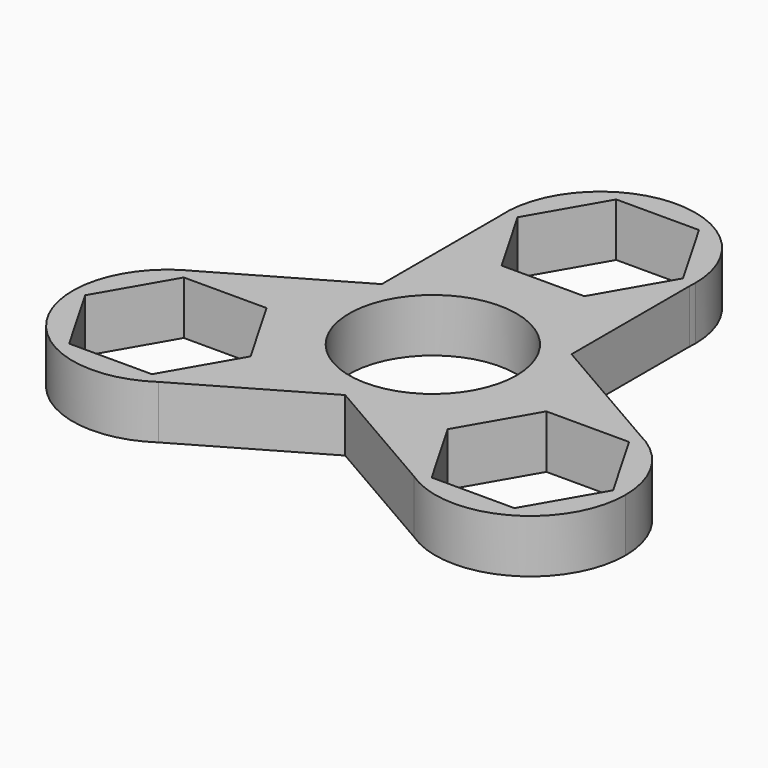
from build123d import *

# Parameters (mm, degrees)
F0_R     = 11
F1_DEPTH = 7
F3_DEPTH = 25


# Not quite as in the source:
# - a feature of the source that left no trace in its solid (it failed there, or was rolled back) is left out
# - a feature names something its author has since deleted; it is built from what else it names


with BuildPart() as f1:
    # F0 (on Top) → F1 (new body)
    with BuildSketch(Plane.XY):
        with BuildLine():
            ThreePointArc((-12.4653791721, 26.5703107531), (0, 15), (12.4653791721, 26.5703107531))
            ThreePointArc((12.4653791721, 26.5703107531), (12.4913417944, 27.0348331758), (12.5, 27.5))
            ThreePointArc((12.5, 27.5), (-0.4651668242, 39.9913417944), (-12.4653791721, 26.5703107531))
        make_face()
        with BuildLine():
            ThreePointArc((12.4653791721, 6.3729366932), (13.6109387701, 3.277551799), (14, 0))
            ThreePointArc((14, 0), (10.1486428448, -9.6439125052), (0.713564513, -13.9818033775))
            Line((0.713564513, -13.9818033775), (0, -14.3937800411))
            Line((0, -14.3937800411), (16.7778745126, -24.0804904074))
            ThreePointArc((16.7778745126, -24.0804904074), (12.9903810568, -7.5), (29.2432536847, -2.4898203457))
            Line((29.2432536847, -2.4898203457), (12.4653791721, 7.1968900206))
            Line((12.4653791721, 7.1968900206), (12.4653791721, 6.3729366932))
        make_face()
        with BuildLine():
            ThreePointArc((-29.2432536847, -2.4898203457), (-34.6410161514, -20), (-16.7778745126, -24.0804904074))
            ThreePointArc((-16.7778745126, -24.0804904074), (-12.7652958706, -19.5928246104), (-11.3156986041, -13.75))
            ThreePointArc((-11.3156986041, -13.75), (-17.1671814201, -3.1647640908), (-29.2432536847, -2.4898203457))
        make_face()
        with BuildLine():
            ThreePointArc((36.3156986041, -13.75), (34.4009345133, -7.101482816), (29.2432536847, -2.4898203457))
            ThreePointArc((29.2432536847, -2.4898203457), (12.9903810568, -7.5), (16.7778745126, -24.0804904074))
            ThreePointArc((16.7778745126, -24.0804904074), (29.6585232145, -24.8004027335), (36.3156986041, -13.75))
        make_face()
        with BuildLine():
            Line((0, -14.3937800411), (-0.713564513, -13.9818033775))
            ThreePointArc((-0.713564513, -13.9818033775), (-12.124355653, -7), (-12.4653791721, 6.3729366932))
            Line((-12.4653791721, 6.3729366932), (-12.4653791721, 7.1968900206))
            Line((-12.4653791721, 7.1968900206), (-29.2432536847, -2.4898203457))
            ThreePointArc((-29.2432536847, -2.4898203457), (-17.1671814201, -3.1647640908), (-11.3156986041, -13.75))
            ThreePointArc((-11.3156986041, -13.75), (-12.7652958706, -19.5928246104), (-16.7778745126, -24.0804904074))
            Line((-16.7778745126, -24.0804904074), (0, -14.3937800411))
        make_face()
        with BuildLine():
            ThreePointArc((0.713564513, -13.9818033775), (10.1486428448, -9.6439125052), (14, 0))
            ThreePointArc((14, 0), (13.6109387701, 3.277551799), (12.4653791721, 6.3729366932))
            ThreePointArc((12.4653791721, 6.3729366932), (12.124355653, 7), (11.7518146591, 7.6088666842))
            ThreePointArc((11.7518146591, 7.6088666842), (0, 14), (-11.7518146591, 7.6088666842))
            ThreePointArc((-11.7518146591, 7.6088666842), (-12.124355653, 7), (-12.4653791721, 6.3729366932))
            ThreePointArc((-12.4653791721, 6.3729366932), (-12.124355653, -7), (-0.713564513, -13.9818033775))
            ThreePointArc((-0.713564513, -13.9818033775), (0, -14), (0.713564513, -13.9818033775))
        make_face()
        Circle(F0_R, mode=Mode.SUBTRACT)
        with BuildLine():
            ThreePointArc((-11.7518146591, 7.6088666842), (0, 14), (11.7518146591, 7.6088666842))
            Line((11.7518146591, 7.6088666842), (12.4653791721, 7.1968900206))
            Line((12.4653791721, 7.1968900206), (12.4653791721, 26.5703107531))
            ThreePointArc((12.4653791721, 26.5703107531), (0, 15), (-12.4653791721, 26.5703107531))
            Line((-12.4653791721, 26.5703107531), (-12.4653791721, 7.1968900206))
            Line((-12.4653791721, 7.1968900206), (-11.7518146591, 7.6088666842))
        make_face()
        with BuildLine():
            ThreePointArc((-12.4653791721, 6.3729366932), (-12.124355653, 7), (-11.7518146591, 7.6088666842))
            Line((-11.7518146591, 7.6088666842), (-12.4653791721, 7.1968900206))
            Line((-12.4653791721, 7.1968900206), (-12.4653791721, 6.3729366932))
        make_face()
        with BuildLine():
            Line((0, -14.3937800411), (0.713564513, -13.9818033775))
            ThreePointArc((0.713564513, -13.9818033775), (0, -14), (-0.713564513, -13.9818033775))
            Line((-0.713564513, -13.9818033775), (0, -14.3937800411))
        make_face()
        with BuildLine():
            ThreePointArc((11.7518146591, 7.6088666842), (12.124355653, 7), (12.4653791721, 6.3729366932))
            Line((12.4653791721, 6.3729366932), (12.4653791721, 7.1968900206))
            Line((12.4653791721, 7.1968900206), (11.7518146591, 7.6088666842))
        make_face()
    extrude(amount=F1_DEPTH)

    # F2 (on face) → F3 (cut)
    with BuildSketch(Plane.XY.offset(7)):
        Polygon((5.4357527844, 36.915), (-5.4357527844, 36.915), (-10.8715055688, 27.5), (-5.4357527844, 18.085), (5.4357527844, 18.085), (10.8715055688, 27.5), align=None)
        Polygon((-18.3799458197, -23.165), (-12.9441930352, -13.75), (-18.3799458197, -4.335), (-29.2514513885, -4.335), (-34.6872041729, -13.75), (-29.2514513885, -23.165), align=None)
        Polygon((29.2514513885, -4.335), (18.3799458197, -4.335), (12.9441930352, -13.75), (18.3799458197, -23.165), (29.2514513885, -23.165), (34.6872041729, -13.75), align=None)
    extrude(amount=-F3_DEPTH, mode=Mode.SUBTRACT)


solid = f1.part
